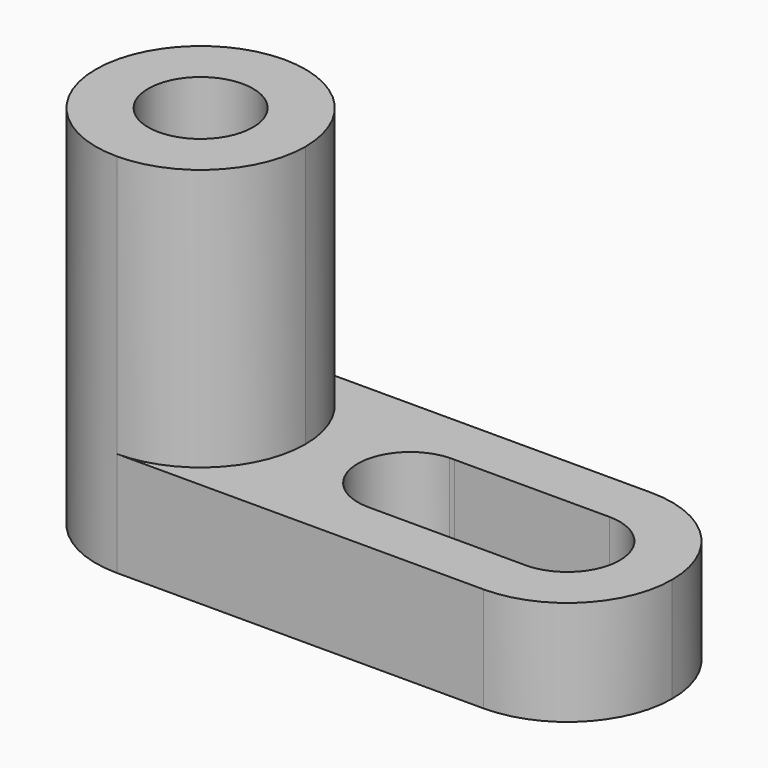
from build123d import *

# Parameters (mm, degrees)
F0_W      = 69.85
F0_H      = 44.45
F1_DEPTH  = 25.4
F2_W      = 44.45
F2_H      = 31.75
F3_DEPTH  = 25.4
F5_DEPTH  = 50.8
F7_DEPTH  = 50.8
F9_DEPTH  = 31.75
F11_DEPTH = 31.75
F13_DEPTH = 25.4
F14_R     = 6.35
F15_DEPTH = 50.8
F17_DEPTH = 25.4


# Not quite as in the source:
# - ends of sketch curves that miss each other by under 0.0002 mm in the source are joined


with BuildPart() as f1:
    # F0 (on Front) → F1 (new body)
    with BuildSketch(Plane.XZ):
        with Locations((34.925, 22.225)):
            Rectangle(F0_W, F0_H)
    extrude(amount=F1_DEPTH)

    # F2 (on face) → F3 (cut)
    with BuildSketch(Plane.XZ.offset(25.4)):
        with Locations((47.625, 28.575)):
            Rectangle(F2_W, F2_H)
    extrude(amount=-F3_DEPTH, mode=Mode.SUBTRACT)

    # F4 (on face) → F5 (cut)
    with BuildSketch(Plane.XY.offset(44.45)):
        with BuildLine():
            ThreePointArc((0, -12.7), (3.7197438789, -3.7197438789), (12.7, 0))
            Line((12.7, 0), (0, 0))
            Line((0, 0), (0, -12.7))
        make_face()
    extrude(amount=-F5_DEPTH, mode=Mode.SUBTRACT)

    # F6 (on face) → F7 (cut)
    with BuildSketch(Plane.XY.offset(44.45)):
        with BuildLine():
            ThreePointArc((12.7, -25.4), (3.7197438789, -21.6802561211), (0, -12.7))
            Line((0, -12.7), (0, -25.4))
            Line((0, -25.4), (12.7, -25.4))
        make_face()
    extrude(amount=-F7_DEPTH, mode=Mode.SUBTRACT)

    # F8 (on face) → F9 (cut)
    with BuildSketch(Plane.XY.offset(44.45)):
        with BuildLine():
            ThreePointArc((25.4, -12.7), (21.6802561211, -21.6802561211), (12.7, -25.4))
            Line((12.7, -25.4), (25.4, -25.4))
            Line((25.4, -25.4), (25.4, -12.7))
        make_face()
    extrude(amount=-F9_DEPTH, mode=Mode.SUBTRACT)

    # F10 (on face) → F11 (cut)
    with BuildSketch(Plane.XY.offset(44.45)):
        with BuildLine():
            ThreePointArc((12.7, 0), (21.6802561211, -3.7197438789), (25.4, -12.7))
            Line((25.4, -12.7), (25.4, 0))
            Line((25.4, 0), (12.7, 0))
        make_face()
    extrude(amount=-F11_DEPTH, mode=Mode.SUBTRACT)

    # F12 (on face) → F13 (cut)
    with BuildSketch(Plane.XY.offset(12.7)):
        with BuildLine():
            ThreePointArc((57.1496006293, -19.0499999874), (50.8, -12.7), (57.1496006293, -6.3500000126))
            Line((57.1496006293, -6.3500000126), (38.3825719247, -6.3562902725))
            ThreePointArc((38.3825719247, -6.3562902725), (42.6889449616, -8.3109130632), (44.45, -12.7))
            ThreePointArc((44.45, -12.7), (42.6333883945, -17.1464468584), (38.2229481372, -19.048809633))
            Line((38.2229481372, -19.048809633), (57.1496006293, -19.0499999874))
        make_face()
        with BuildLine():
            ThreePointArc((57.1496006293, -19.0499999874), (61.6399868594, -17.1902692572), (63.5, -12.7))
            ThreePointArc((63.5, -12.7), (61.6399868594, -8.2097307428), (57.1496006293, -6.3500000126))
            ThreePointArc((57.1496006293, -6.3500000126), (50.8, -12.7), (57.1496006293, -19.0499999874))
        make_face()
        with BuildLine():
            Line((37.81317546, -6.3564811277), (38.3825719247, -6.3562902725))
            ThreePointArc((38.3825719247, -6.3562902725), (38.0978715521, -6.3500003567), (37.81317546, -6.3564811277))
        make_face()
        with BuildLine():
            ThreePointArc((44.45, -12.7), (42.6889449616, -8.3109130632), (38.3825719247, -6.3562902725))
            Line((38.3825719247, -6.3562902725), (37.81317546, -6.3564811277))
            ThreePointArc((37.81317546, -6.3564811277), (31.7505240807, -12.7815815558), (37.9762532721, -19.0487941176))
            Line((37.9762532721, -19.0487941176), (38.2229481372, -19.048809633))
            ThreePointArc((38.2229481372, -19.048809633), (42.6333883945, -17.1464468584), (44.45, -12.7))
        make_face()
        with BuildLine():
            ThreePointArc((37.9762532721, -19.0487941176), (38.0996006293, -19.0499999874), (38.2229481372, -19.048809633))
            Line((38.2229481372, -19.048809633), (37.9762532721, -19.0487941176))
        make_face()
    extrude(amount=-F13_DEPTH, mode=Mode.SUBTRACT)

    # F14 (on face) → F15 (cut)
    with BuildSketch(Plane.XY.offset(44.45)):
        with Locations((12.7, -12.7)):
            Circle(F14_R)
    extrude(amount=-F15_DEPTH, mode=Mode.SUBTRACT)

    # F16 (on face) → F17 (cut)
    with BuildSketch(Plane.XY.offset(12.7)):
        with BuildLine():
            Line((69.85, -25.4), (69.85, -12.7))
            ThreePointArc((69.85, -12.7), (66.1302561211, -21.6802561211), (57.15, -25.4))
            Line((57.15, -25.4), (69.85, -25.4))
        make_face()
        with BuildLine():
            ThreePointArc((57.15, 0), (66.1302561211, -3.7197438789), (69.85, -12.7))
            Line((69.85, -12.7), (69.85, 0))
            Line((69.85, 0), (57.15, 0))
        make_face()
    extrude(amount=-F17_DEPTH, mode=Mode.SUBTRACT)


solid = f1.part
